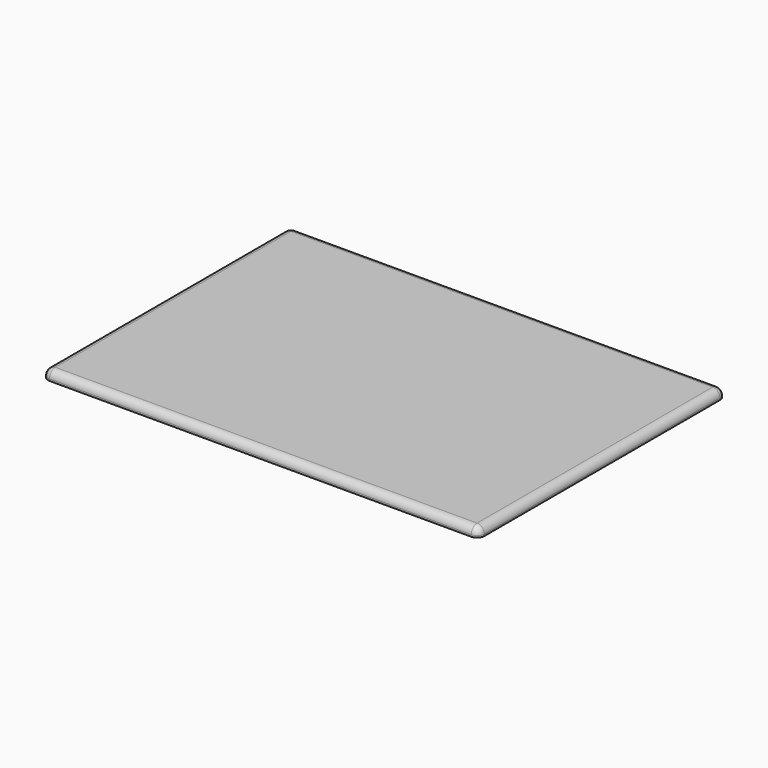
from build123d import *

# Parameters (mm, degrees)
F0_W         = 304.8
F0_H         = 215.9
F1_DEPTH     = 6.35
F2_R         = 5.08
F3_T1_DEPTH  = 13.97
F3_S5_W      = 5.08
F3_S5_H      = 5.08
F3_T6_DEPTH  = 5.08
F3_S11_W     = 5.08
F3_S11_H     = 5.08
F3_T12_DEPTH = 5.08
F3_S17_W     = 5.08
F3_S17_H     = 5.08
F3_T18_DEPTH = 5.08


# Not quite as in the source:
# - a fillet or chamfer that OpenCascade refuses, or shapes differently, is made with other operations: its cross-section is extruded or revolved along the edge and cut away or added


with BuildPart() as f1:
    # F0 (on Top) → F1 (new body)
    with BuildSketch(Plane.XY):
        with Locations((0.3756433725, 24.0940256725)):
            Rectangle(F0_W, F0_H)
    extrude(amount=F1_DEPTH)

    # F2
    f2_edges = [f1.edges().sort_by_distance(p)[0] for p in [
        (152.775643, -83.855974, 3.175),
        (0.375643, -83.855974, 6.35),
        (-152.024357, 24.094026, 6.35),
        (0.375643, 132.044026, 6.35),
        (152.775643, 24.094026, 6.35),
    ]]
    fillet(f2_edges, radius=F2_R)

    # F3: fillet of radius 5.08 on 3 edges, made by hand

    # F3_s2 → F3_t1 (cut)
    with BuildSketch(Plane.XY.offset(-12.7)):
        with BuildLine():
            ThreePointArc((-152.0243566275, -78.7759743275), (-150.5364590759, -82.3680767759), (-146.9443566275, -83.8559743275))
            Line((-146.9443566275, -83.8559743275), (-152.0243566275, -83.8559743275))
            Line((-152.0243566275, -83.8559743275), (-152.0243566275, -78.7759743275))
        make_face()
        with BuildLine():
            ThreePointArc((-146.9443566275, 132.0440256725), (-150.5364590759, 130.556128121), (-152.0243566275, 126.9640256725))
            Line((-152.0243566275, 126.9640256725), (-152.0243566275, 132.0440256725))
            Line((-152.0243566275, 132.0440256725), (-146.9443566275, 132.0440256725))
        make_face()
        with BuildLine():
            ThreePointArc((152.7756433725, 126.9640256725), (151.287745821, 130.556128121), (147.6956433725, 132.0440256725))
            Line((147.6956433725, 132.0440256725), (152.7756433725, 132.0440256725))
            Line((152.7756433725, 132.0440256725), (152.7756433725, 126.9640256725))
        make_face()
    extrude(amount=F3_T1_DEPTH, mode=Mode.SUBTRACT)


with BuildPart() as f3_tool4:
    # F3_s5 → F3_t6 (new body)
    with BuildSketch(Plane.YZ.offset(147.6956433725)):
        with Locations((129.5040256725, 3.81)):
            Rectangle(F3_S5_W, F3_S5_H)
    extrude(amount=F3_T6_DEPTH)

    # F3_s7 → F3_t8 (revolve, cut)
    with BuildSketch(Plane(origin=(147.6956433725, 126.9640256725, 1.27), x_dir=(0, -0.7071067812, -0.7071067812), z_dir=(0, -0.7071067812, 0.7071067812))):
        with BuildLine():
            ThreePointArc((0, -5.08), (5.08, 0), (0, 5.08))
            Line((0, 5.08), (0, -5.08))
        make_face()
    revolve(axis=Axis((147.6956433725, 126.9640256725, 1.27), (1, 0, 0)), mode=Mode.SUBTRACT)


with BuildPart() as f1_1:
    add(f1.part)

    # F3_t3: cut F3_tool4
    add(f3_tool4.part, mode=Mode.SUBTRACT)


with BuildPart() as f3_tool10:
    # F3_s11 → F3_t12 (new body)
    with BuildSketch(Plane.XZ.offset(-126.9640256725)):
        with Locations((-149.4843566275, 3.81)):
            Rectangle(F3_S11_W, F3_S11_H)
    extrude(amount=-F3_T12_DEPTH)

    # F3_s13 → F3_t14 (revolve, cut)
    with BuildSketch(Plane(origin=(-146.9443566275, 126.9640256725, 1.27), x_dir=(0.7071067812, 0, -0.7071067812), z_dir=(0.7071067812, 0, 0.7071067812))):
        with BuildLine():
            ThreePointArc((0, -5.08), (5.08, 0), (0, 5.08))
            Line((0, 5.08), (0, -5.08))
        make_face()
    revolve(axis=Axis((-146.9443566275, 126.9640256725, 1.27), (0, 1, 0)), mode=Mode.SUBTRACT)


with BuildPart() as f1_2:
    add(f1_1.part)

    # F3_t9: cut F3_tool10
    add(f3_tool10.part, mode=Mode.SUBTRACT)


with BuildPart() as f3_tool16:
    # F3_s17 → F3_t18 (new body)
    with BuildSketch(Plane.YZ.offset(-146.9443566275)):
        with Locations((-81.3159743275, 3.81)):
            Rectangle(F3_S17_W, F3_S17_H)
    extrude(amount=-F3_T18_DEPTH)

    # F3_s19 → F3_t20 (revolve, cut)
    with BuildSketch(Plane(origin=(-146.9443566275, -78.7759743275, 1.27), x_dir=(0, 0.7071067812, -0.7071067812), z_dir=(0, 0.7071067812, 0.7071067812))):
        with BuildLine():
            ThreePointArc((0, -5.08), (5.08, 0), (0, 5.08))
            Line((0, 5.08), (0, -5.08))
        make_face()
    revolve(axis=Axis((-146.9443566275, -78.7759743275, 1.27), (-1, 0, 0)), mode=Mode.SUBTRACT)


with BuildPart() as f1_3:
    add(f1_2.part)

    # F3_t15: cut F3_tool16
    add(f3_tool16.part, mode=Mode.SUBTRACT)


solid = f1_3.part
